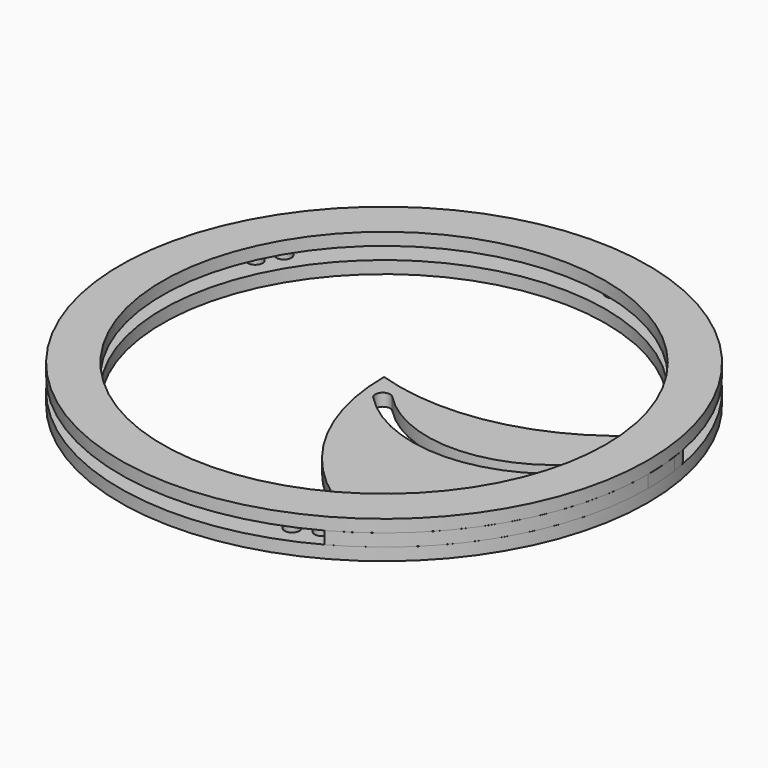
from build123d import *

# Parameters (mm, degrees)
F1_R          = 1.5
F2_DEPTH      = 2.5
F3_R          = 53.1009930313
F3_R_2        = 1.5
F3_R_3        = 44.5707546786
F4_DEPTH      = 2.5
F5_DEPTH      = 2.5
F6_R          = 53.1009930313
F6_R_2        = 1.5
F6_R_3        = 44.5707546786
F7_DEPTH      = 2.5
F8_DEPTH      = 2.5
F8_DEPTH_BACK = 2.5


with BuildPart() as f2:
    # F1 (on Top) → F2 (new body)
    with BuildSketch(Plane.XY):
        with BuildLine():
            ThreePointArc((43.5967767518, 9.2667809662), (23.0399016141, -1.2074700785), (0, 0))
            ThreePointArc((0, 0), (5.9713488611, -22.2853773393), (22.2853773393, -38.5994058175))
            Line((22.2853773393, -38.5994058175), (23.1836535337, -39.1180258202))
            ThreePointArc((23.1836535337, -39.1180258202), (26.5451077793, -42.2431398769), (25.3313187663, -46.6694734325))
            ThreePointArc((25.3313187663, -46.6694734325), (45.6335054658, -27.1532436334), (53.1009930313, 0))
            ThreePointArc((53.1009930313, 0), (52.977739866, 3.6158732827), (52.6085525382, 7.2149608971))
            ThreePointArc((52.6085525382, 7.2149608971), (52.4252049406, 8.4447230767), (52.2131148088, 9.6698553699))
            ThreePointArc((52.2131148088, 9.6698553699), (48.3785028701, 12.1920496116), (44.3675962945, 9.96083))
            Line((44.3675962945, 9.96083), (43.5967767518, 9.2667809662))
        make_face()
        with BuildLine():
            ThreePointArc((50.1306670439, 2.3607243834), (49.5983825966, 1.1676379558), (49.0123761454, 0))
            ThreePointArc((49.0123761454, 0), (27.6850730752, -14.9678218042), (3.035185807, -6.5255114881))
            ThreePointArc((3.035185807, -6.5255114881), (3.0681178737, -4.404446784), (5.1891825778, -4.4373788507))
            ThreePointArc((5.1891825778, -4.4373788507), (26.4597740482, -12.0987734107), (45.5583266127, 0))
            ThreePointArc((45.5583266127, 0), (46.5289054338, 1.7254070276), (47.3638609946, 3.5203727292))
            ThreePointArc((47.3638609946, 3.5203727292), (49.0429796454, 4.411110445), (50.2472640193, 2.9405485563))
            ThreePointArc((50.2472640193, 2.9405485563), (50.2178259079, 2.6448329302), (50.1306670439, 2.3607243834))
        make_face(mode=Mode.SUBTRACT)
        with Locations((48.2143656672, 7.7664353785)):
            Circle(F1_R, mode=Mode.SUBTRACT)
    extrude(amount=F2_DEPTH)


with BuildPart() as f4:
    # F3 (on Top) → F4 (new body)
    with BuildSketch(Plane.XY):
        Circle(F3_R)
        with Locations((-34.4412450194, -34.6228712947)):
            Circle(F3_R_2, mode=Mode.SUBTRACT)
        with Locations((22.2853773393, -43.4546261291)):
            Circle(F3_R_2, mode=Mode.SUBTRACT)
        with Locations((-43.5712373761, 22.0565148808)):
            Circle(F3_R_2, mode=Mode.SUBTRACT)
        Circle(F3_R_3, mode=Mode.SUBTRACT)
        with Locations((48.2143656672, 7.7664353785)):
            Circle(F3_R_2, mode=Mode.SUBTRACT)
        with Locations((7.512739389, 48.2545471645)):
            Circle(F3_R_2, mode=Mode.SUBTRACT)
        with Locations((22.2853773393, -43.4546261291)):
            Circle(F3_R_2)
        with Locations((48.2143656672, 7.7664353785)):
            Circle(F3_R_2)
        with Locations((7.512739389, 48.2545471645)):
            Circle(F3_R_2)
        with Locations((-43.5712373761, 22.0565148808)):
            Circle(F3_R_2)
        with Locations((-34.4412450194, -34.6228712947)):
            Circle(F3_R_2)
    extrude(amount=-F4_DEPTH)

    # F3 (on Top) → F5 (join)
    with BuildSketch(Plane.XY):
        with Locations((7.512739389, 48.2545471645)):
            Circle(F3_R_2)
        with Locations((-43.5712373761, 22.0565148808)):
            Circle(F3_R_2)
        with Locations((-34.4412450194, -34.6228712947)):
            Circle(F3_R_2)
        with Locations((22.2853773393, -43.4546261291)):
            Circle(F3_R_2)
        with Locations((48.2143656672, 7.7664353785)):
            Circle(F3_R_2)
    extrude(amount=F5_DEPTH)


with BuildPart() as f7:
    # F6 (on face) → F7 (new body)
    with BuildSketch(Plane.XY.offset(2.5)):
        Circle(F6_R)
        with Locations((-37.7089539458, -31.031876635)):
            Circle(F6_R_2, mode=Mode.SUBTRACT)
        with Locations((17.8603608772, -45.4527236204)):
            Circle(F6_R_2, mode=Mode.SUBTRACT)
        with Locations((-41.1657760959, 26.2739691253)):
            Circle(F6_R_2, mode=Mode.SUBTRACT)
        Circle(F6_R_3, mode=Mode.SUBTRACT)
        with Locations((48.7472640193, 2.9405485563)):
            Circle(F6_R_2, mode=Mode.SUBTRACT)
        with Locations((12.2671051452, 47.2700825738)):
            Circle(F6_R_2, mode=Mode.SUBTRACT)
    extrude(amount=F7_DEPTH)

    # F6 (on face) → F8 (join, two sides)
    with BuildSketch(Plane.XY.offset(2.5)) as f8_sk:
        with Locations((-37.7089539458, -31.031876635)):
            Circle(F6_R_2)
        with Locations((-41.1657760959, 26.2739691253)):
            Circle(F6_R_2)
        with Locations((12.2671051452, 47.2700825738)):
            Circle(F6_R_2)
        with BuildLine():
            ThreePointArc((50.1306670439, 2.3607243834), (50.2178259079, 2.6448329302), (50.2472640193, 2.9405485563))
            ThreePointArc((50.2472640193, 2.9405485563), (49.0429796454, 4.411110445), (47.3638609946, 3.5203727292))
            ThreePointArc((47.3638609946, 3.5203727292), (48.1674398464, 1.5571455317), (50.1306670439, 2.3607243834))
        make_face()
        with Locations((17.8603608772, -45.4527236204)):
            Circle(F6_R_2)
    extrude(amount=-F8_DEPTH)
    extrude(f8_sk.sketch, amount=F8_DEPTH_BACK)


solid = Compound([f2.part, f4.part, f7.part])
